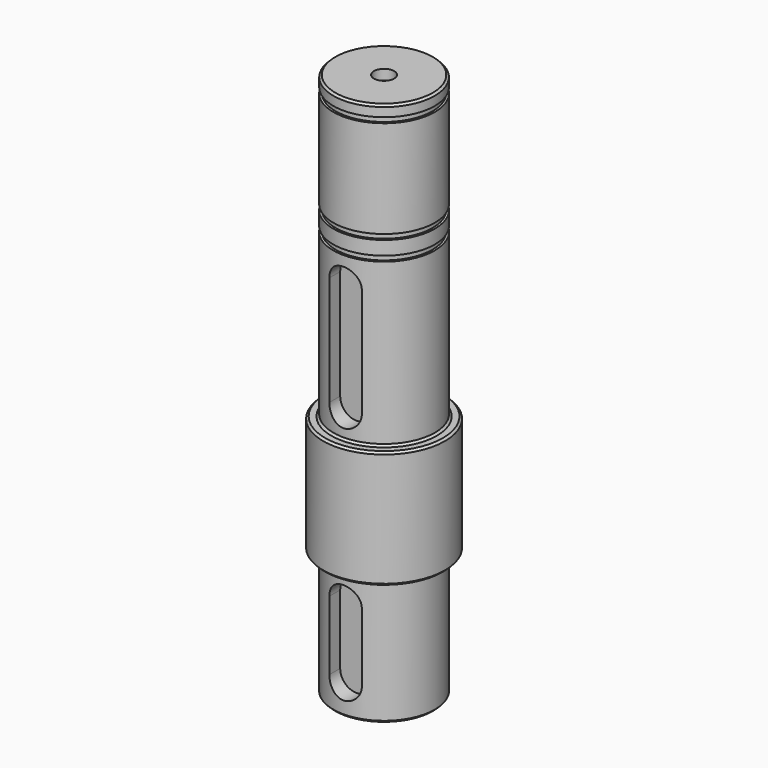
from build123d import *

# Parameters (mm, degrees)
F2_SIZE  = 0.5
F5_DEPTH = 25


with BuildPart() as f1:
    # F0 (on Front) → F1 (revolve)
    with BuildSketch(Plane.XZ):
        Polygon((0, 23), (0, 0), (0, -101), (2.5, -103.5), (2.5, -106), (12.5, -106), (12.5, -105), (12.5, -75), (15, -75), (15, -51), (15, -46), (12.5, -46), (12.5, -6), (11.95, -6), (11.95, -4.7), (12.5, -4.7), (12.5, -1.3), (11.95, -1.3), (11.95, 0), (12.5, 0), (12.5, 24), (11.95, 24), (11.95, 25.3), (12.475, 25.3), (12.475, 28), (2.5, 28), (2.5, 25.5), align=None)
    revolve(axis=Axis((0, 0, -50.5), (0, 0, 1)))

    # F2
    f2_edges = [f1.edges().sort_by_distance(p)[0] for p in [
        (-15, 0, -46),
        (-12.5, 0, -46),
        (-12.5, 0, -75),
        (-15, 0, -75),
        (-12.475, 0, 28),
        (-2.5, 0, -106),
        (-12.5, 0, -106),
    ]]
    chamfer(f2_edges, length=F2_SIZE)

    # F4 (on offset) → F5 (cut)
    with BuildSketch(Plane.XZ.offset(8.5)):
        with BuildLine():
            ThreePointArc((-4, -39.5), (0, -43.5), (4, -39.5))
            Line((4, -39.5), (4, -12.5))
            ThreePointArc((4, -12.5), (0, -8.5), (-4, -12.5))
            Line((-4, -12.5), (-4, -39.5))
        make_face()
        with BuildLine():
            Line((4, -98.5), (4, -81.5))
            ThreePointArc((4, -81.5), (0, -77.5), (-4, -81.5))
            Line((-4, -81.5), (-4, -98.5))
            ThreePointArc((-4, -98.5), (0, -102.5), (4, -98.5))
        make_face()
    extrude(amount=F5_DEPTH, mode=Mode.SUBTRACT)


solid = f1.part
